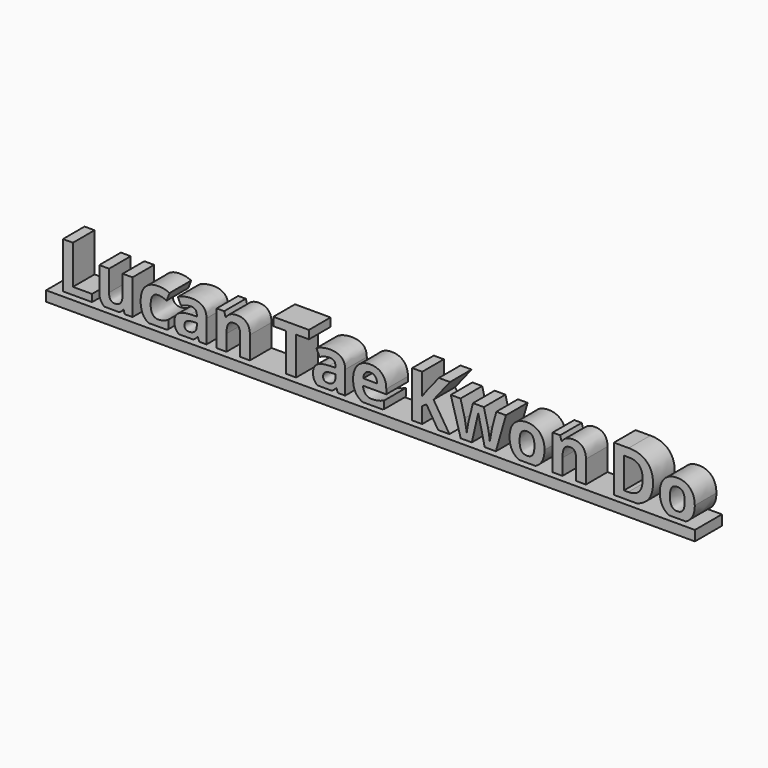
from build123d import *

# Parameters (mm, degrees)
F0_TEXT_SIZE = 9.7667544818
F1_DEPTH     = 4
F2_W         = 96
F2_H         = 1.5
F3_DEPTH     = 5


# Not quite as in the source:
# - Text() gives the source's letters only with a copy of the font that has no kerning and outlines rounded to 1/6400 em; it was checked with that copy


with BuildPart() as f1:
    # F0 (on Front) → F1 (new body)
    with BuildSketch(Plane.XZ):
        with Locations((-35.3357957374, 7.4166220276)):
            Text('Lucan Tae Kwon Do', F0_TEXT_SIZE, font='Open Sans', font_style=FontStyle.BOLD, text_align=(TextAlign.LEFT, TextAlign.BOTTOM))
    extrude(amount=F1_DEPTH)

    # F2 (on Front) → F3 (join)
    with BuildSketch(Plane.XZ):
        with Locations((11.8476489731, 6.8208258599)):
            Rectangle(F2_W, F2_H)
    extrude(amount=F3_DEPTH)


solid = f1.part
